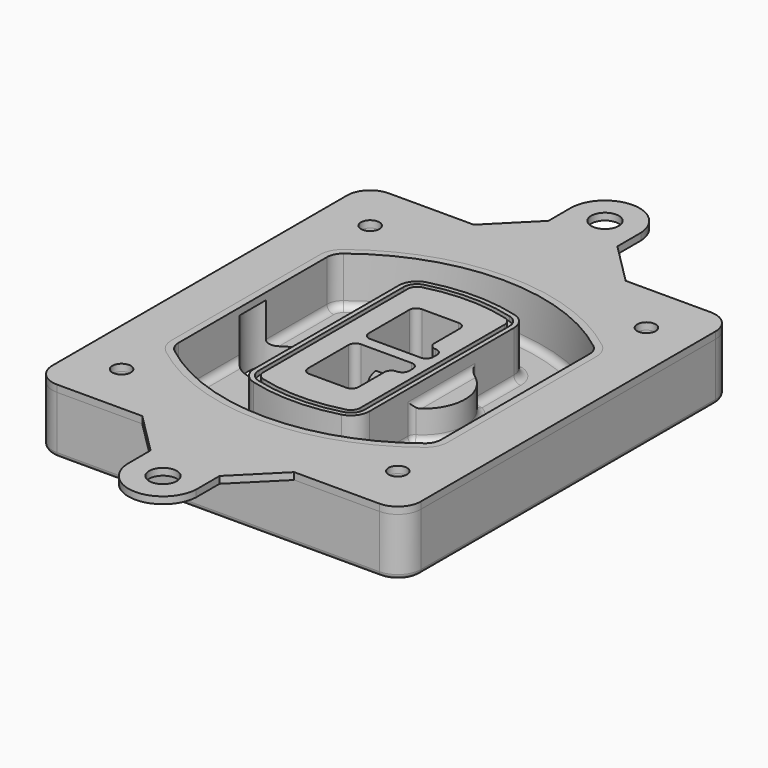
from build123d import *

# Parameters (mm, degrees)
F0_R      = 4
F1_DEPTH  = 25
F2_DEPTH  = 3
F3_DEPTH  = 18
F5_DEPTH  = 21
F6_DEPTH  = 2
F8_DEPTH  = 20
F9_DEPTH  = 16
F10_DEPTH = 25
F7_R      = 6
F7_R_2    = 4
F11_DEPTH = 6
F13_DEPTH = 9
F14_R     = 3
F15_R     = 2
F16_R     = 6
F16_R_2   = 4
F17_DEPTH = 3


with BuildPart() as f1:
    # F0 (on Top) → F1 (new body)
    with BuildSketch(Plane.XY):
        with BuildLine():
            ThreePointArc((-80, -80), (-77.0710678119, -87.0710678119), (-70, -90))
            Line((-70, -90), (70, -90))
            ThreePointArc((70, -90), (77.0710678119, -87.0710678119), (80, -80))
            Line((80, -80), (80, 80))
            ThreePointArc((80, 80), (77.0710678119, 87.0710678119), (70, 90))
            Line((70, 90), (-70, 90))
            ThreePointArc((-70, 90), (-77.0710678119, 87.0710678119), (-80, 80))
            Line((-80, 80), (-80, -80))
        make_face()
        with Locations((-60, -67.5)):
            Circle(F0_R, mode=Mode.SUBTRACT)
        with Locations((60, -67.5)):
            Circle(F0_R, mode=Mode.SUBTRACT)
        with Locations((-60, 67.5)):
            Circle(F0_R, mode=Mode.SUBTRACT)
        with BuildLine():
            ThreePointArc((-64, 40.2934422872), (-62.5820384798, 46.4328484224), (-58.6153846154, 51.3286200352))
            ThreePointArc((-58.6153846154, 51.3286200352), (0, 71.5), (58.6153846154, 51.3286200352))
            ThreePointArc((58.6153846154, 51.3286200352), (62.5820384798, 46.4328484224), (64, 40.2934422872))
            Line((64, 40.2934422872), (64, -40.2934422872))
            ThreePointArc((64, -40.2934422872), (62.5820384798, -46.4328484224), (58.6153846154, -51.3286200352))
            ThreePointArc((58.6153846154, -51.3286200352), (0, -71.5), (-58.6153846154, -51.3286200352))
            ThreePointArc((-58.6153846154, -51.3286200352), (-62.5820384798, -46.4328484224), (-64, -40.2934422872))
            Line((-64, -40.2934422872), (-64, 40.2934422872))
        make_face(mode=Mode.SUBTRACT)
        with Locations((60, 67.5)):
            Circle(F0_R, mode=Mode.SUBTRACT)
        with BuildLine():
            ThreePointArc((58.6153846154, 51.3286200352), (0, 71.5), (-58.6153846154, 51.3286200352))
            ThreePointArc((-58.6153846154, 51.3286200352), (-62.5820384798, 46.4328484224), (-64, 40.2934422872))
            Line((-64, 40.2934422872), (-64, -40.2934422872))
            ThreePointArc((-64, -40.2934422872), (-62.5820384798, -46.4328484224), (-58.6153846154, -51.3286200352))
            ThreePointArc((-58.6153846154, -51.3286200352), (0, -71.5), (58.6153846154, -51.3286200352))
            ThreePointArc((58.6153846154, -51.3286200352), (62.5820384798, -46.4328484224), (64, -40.2934422872))
            Line((64, -40.2934422872), (64, 40.2934422872))
            ThreePointArc((64, 40.2934422872), (62.5820384798, 46.4328484224), (58.6153846154, 51.3286200352))
        make_face()
        with BuildLine():
            Line((-60, -40.2934422872), (-60, 40.2934422872))
            ThreePointArc((-60, 40.2934422872), (-58.9871703427, 44.6787323838), (-56.1538461538, 48.1757121072))
            ThreePointArc((-56.1538461538, 48.1757121072), (0, 67.5), (56.1538461538, 48.1757121072))
            ThreePointArc((56.1538461538, 48.1757121072), (58.9871703427, 44.6787323838), (60, 40.2934422872))
            Line((60, 40.2934422872), (60, -40.2934422872))
            ThreePointArc((60, -40.2934422872), (58.9871703427, -44.6787323838), (56.1538461538, -48.1757121072))
            ThreePointArc((56.1538461538, -48.1757121072), (0, -67.5), (-56.1538461538, -48.1757121072))
            ThreePointArc((-56.1538461538, -48.1757121072), (-58.9871703427, -44.6787323838), (-60, -40.2934422872))
        make_face(mode=Mode.SUBTRACT)
        with BuildLine():
            ThreePointArc((-56.1538461538, 48.1757121072), (-58.9871703427, 44.6787323838), (-60, 40.2934422872))
            Line((-60, 40.2934422872), (-60, -40.2934422872))
            ThreePointArc((-60, -40.2934422872), (-58.9871703427, -44.6787323838), (-56.1538461538, -48.1757121072))
            ThreePointArc((-56.1538461538, -48.1757121072), (0, -67.5), (56.1538461538, -48.1757121072))
            ThreePointArc((56.1538461538, -48.1757121072), (58.9871703427, -44.6787323838), (60, -40.2934422872))
            Line((60, -40.2934422872), (60, 40.2934422872))
            ThreePointArc((60, 40.2934422872), (58.9871703427, 44.6787323838), (56.1538461538, 48.1757121072))
            ThreePointArc((56.1538461538, 48.1757121072), (0, 67.5), (-56.1538461538, 48.1757121072))
        make_face()
        with BuildLine():
            ThreePointArc((54.3076923077, 45.8110311612), (56.2910192399, 43.3631453548), (57, 40.2934422872))
            Line((57, 40.2934422872), (57, -40.2934422872))
            ThreePointArc((57, -40.2934422872), (56.2910192399, -43.3631453548), (54.3076923077, -45.8110311612))
            ThreePointArc((54.3076923077, -45.8110311612), (0, -64.5), (-54.3076923077, -45.8110311612))
            ThreePointArc((-54.3076923077, -45.8110311612), (-56.2910192399, -43.3631453548), (-57, -40.2934422872))
            Line((-57, -40.2934422872), (-57, 40.2934422872))
            ThreePointArc((-57, 40.2934422872), (-56.2910192399, 43.3631453548), (-54.3076923077, 45.8110311612))
            ThreePointArc((-54.3076923077, 45.8110311612), (0, 64.5), (54.3076923077, 45.8110311612))
        make_face(mode=Mode.SUBTRACT)
        with BuildLine():
            Line((57, -40.2934422872), (57, 40.2934422872))
            ThreePointArc((57, 40.2934422872), (56.2910192399, 43.3631453548), (54.3076923077, 45.8110311612))
            ThreePointArc((54.3076923077, 45.8110311612), (0, 64.5), (-54.3076923077, 45.8110311612))
            ThreePointArc((-54.3076923077, 45.8110311612), (-56.2910192399, 43.3631453548), (-57, 40.2934422872))
            Line((-57, 40.2934422872), (-57, -40.2934422872))
            ThreePointArc((-57, -40.2934422872), (-56.2910192399, -43.3631453548), (-54.3076923077, -45.8110311612))
            ThreePointArc((-54.3076923077, -45.8110311612), (0, -64.5), (54.3076923077, -45.8110311612))
            ThreePointArc((54.3076923077, -45.8110311612), (56.2910192399, -43.3631453548), (57, -40.2934422872))
        make_face()
    extrude(amount=-F1_DEPTH)

    # F0 (on Top) → F2 (join)
    with BuildSketch(Plane.XY):
        with BuildLine():
            ThreePointArc((-56.1538461538, 48.1757121072), (-58.9871703427, 44.6787323838), (-60, 40.2934422872))
            Line((-60, 40.2934422872), (-60, -40.2934422872))
            ThreePointArc((-60, -40.2934422872), (-58.9871703427, -44.6787323838), (-56.1538461538, -48.1757121072))
            ThreePointArc((-56.1538461538, -48.1757121072), (0, -67.5), (56.1538461538, -48.1757121072))
            ThreePointArc((56.1538461538, -48.1757121072), (58.9871703427, -44.6787323838), (60, -40.2934422872))
            Line((60, -40.2934422872), (60, 40.2934422872))
            ThreePointArc((60, 40.2934422872), (58.9871703427, 44.6787323838), (56.1538461538, 48.1757121072))
            ThreePointArc((56.1538461538, 48.1757121072), (0, 67.5), (-56.1538461538, 48.1757121072))
        make_face()
        with BuildLine():
            ThreePointArc((54.3076923077, 45.8110311612), (56.2910192399, 43.3631453548), (57, 40.2934422872))
            Line((57, 40.2934422872), (57, -40.2934422872))
            ThreePointArc((57, -40.2934422872), (56.2910192399, -43.3631453548), (54.3076923077, -45.8110311612))
            ThreePointArc((54.3076923077, -45.8110311612), (0, -64.5), (-54.3076923077, -45.8110311612))
            ThreePointArc((-54.3076923077, -45.8110311612), (-56.2910192399, -43.3631453548), (-57, -40.2934422872))
            Line((-57, -40.2934422872), (-57, 40.2934422872))
            ThreePointArc((-57, 40.2934422872), (-56.2910192399, 43.3631453548), (-54.3076923077, 45.8110311612))
            ThreePointArc((-54.3076923077, 45.8110311612), (0, 64.5), (54.3076923077, 45.8110311612))
        make_face(mode=Mode.SUBTRACT)
    extrude(amount=F2_DEPTH)

    # F0 (on Top) → F3 (cut)
    with BuildSketch(Plane.XY):
        with BuildLine():
            Line((57, -40.2934422872), (57, 40.2934422872))
            ThreePointArc((57, 40.2934422872), (56.2910192399, 43.3631453548), (54.3076923077, 45.8110311612))
            ThreePointArc((54.3076923077, 45.8110311612), (0, 64.5), (-54.3076923077, 45.8110311612))
            ThreePointArc((-54.3076923077, 45.8110311612), (-56.2910192399, 43.3631453548), (-57, 40.2934422872))
            Line((-57, 40.2934422872), (-57, -40.2934422872))
            ThreePointArc((-57, -40.2934422872), (-56.2910192399, -43.3631453548), (-54.3076923077, -45.8110311612))
            ThreePointArc((-54.3076923077, -45.8110311612), (0, -64.5), (54.3076923077, -45.8110311612))
            ThreePointArc((54.3076923077, -45.8110311612), (56.2910192399, -43.3631453548), (57, -40.2934422872))
        make_face()
    extrude(amount=-F3_DEPTH, mode=Mode.SUBTRACT)

    # F4 (on face) → F5 (join, through all)
    with BuildSketch(Plane.XY.offset(3)):
        with BuildLine():
            ThreePointArc((-25, -39.2465276821), (-23.3511545998, -44.1109737193), (-19.0842911877, -46.9702398883))
            ThreePointArc((-19.0842911877, -46.9702398883), (0, -49.5), (19.0842911877, -46.9702398883))
            ThreePointArc((19.0842911877, -46.9702398883), (23.3511545998, -44.1109737193), (25, -39.2465276821))
            Line((25, -39.2465276821), (25, 39.2465276821))
            ThreePointArc((25, 39.2465276821), (23.3511545998, 44.1109737193), (19.0842911877, 46.9702398883))
            ThreePointArc((19.0842911877, 46.9702398883), (0, 49.5), (-19.0842911877, 46.9702398883))
            ThreePointArc((-19.0842911877, 46.9702398883), (-23.3511545998, 44.1109737193), (-25, 39.2465276821))
            Line((-25, 39.2465276821), (-25, -39.2465276821))
        make_face()
        with BuildLine():
            ThreePointArc((18.5632183908, 45.0393118368), (21.7633659499, 42.89486221), (23, 39.2465276821))
            Line((23, 39.2465276821), (23, -39.2465276821))
            ThreePointArc((23, -39.2465276821), (21.7633659499, -42.89486221), (18.5632183908, -45.0393118368))
            ThreePointArc((18.5632183908, -45.0393118368), (0, -47.5), (-18.5632183908, -45.0393118368))
            ThreePointArc((-18.5632183908, -45.0393118368), (-21.7633659499, -42.89486221), (-23, -39.2465276821))
            Line((-23, -39.2465276821), (-23, 39.2465276821))
            ThreePointArc((-23, 39.2465276821), (-21.7633659499, 42.89486221), (-18.5632183908, 45.0393118368))
            ThreePointArc((-18.5632183908, 45.0393118368), (0, 47.5), (18.5632183908, 45.0393118368))
        make_face(mode=Mode.SUBTRACT)
        with BuildLine():
            Line((23, -39.2465276821), (23, 39.2465276821))
            ThreePointArc((23, 39.2465276821), (21.7633659499, 42.89486221), (18.5632183908, 45.0393118368))
            ThreePointArc((18.5632183908, 45.0393118368), (0, 47.5), (-18.5632183908, 45.0393118368))
            ThreePointArc((-18.5632183908, 45.0393118368), (-21.7633659499, 42.89486221), (-23, 39.2465276821))
            Line((-23, 39.2465276821), (-23, -39.2465276821))
            ThreePointArc((-23, -39.2465276821), (-21.7633659499, -42.89486221), (-18.5632183908, -45.0393118368))
            ThreePointArc((-18.5632183908, -45.0393118368), (0, -47.5), (18.5632183908, -45.0393118368))
            ThreePointArc((18.5632183908, -45.0393118368), (21.7633659499, -42.89486221), (23, -39.2465276821))
        make_face()
        with BuildLine():
            ThreePointArc((18.0421455939, 43.1083837852), (20.1755772999, 41.6787507007), (21, 39.2465276821))
            Line((21, 39.2465276821), (21, -39.2465276821))
            ThreePointArc((21, -39.2465276821), (20.1755772999, -41.6787507007), (18.0421455939, -43.1083837852))
            ThreePointArc((18.0421455939, -43.1083837852), (0, -45.5), (-18.0421455939, -43.1083837852))
            ThreePointArc((-18.0421455939, -43.1083837852), (-20.1755772999, -41.6787507007), (-21, -39.2465276821))
            Line((-21, -39.2465276821), (-21, 39.2465276821))
            ThreePointArc((-21, 39.2465276821), (-20.1755772999, 41.6787507007), (-18.0421455939, 43.1083837852))
            ThreePointArc((-18.0421455939, 43.1083837852), (0, 45.5), (18.0421455939, 43.1083837852))
        make_face(mode=Mode.SUBTRACT)
        with BuildLine():
            Line((21, -39.2465276821), (21, 39.2465276821))
            ThreePointArc((21, 39.2465276821), (20.1755772999, 41.6787507007), (18.0421455939, 43.1083837852))
            ThreePointArc((18.0421455939, 43.1083837852), (0, 45.5), (-18.0421455939, 43.1083837852))
            ThreePointArc((-18.0421455939, 43.1083837852), (-20.1755772999, 41.6787507007), (-21, 39.2465276821))
            Line((-21, 39.2465276821), (-21, -39.2465276821))
            ThreePointArc((-21, -39.2465276821), (-20.1755772999, -41.6787507007), (-18.0421455939, -43.1083837852))
            ThreePointArc((-18.0421455939, -43.1083837852), (0, -45.5), (18.0421455939, -43.1083837852))
            ThreePointArc((18.0421455939, -43.1083837852), (20.1755772999, -41.6787507007), (21, -39.2465276821))
        make_face()
        with BuildLine():
            Line((-8, -2.5), (14, -2.5))
            ThreePointArc((14, -2.5), (16.1213203436, -3.3786796564), (17, -5.5))
            Line((17, -5.5), (17, -7.5))
            ThreePointArc((17, -7.5), (16.1213203436, -9.6213203436), (14, -10.5))
            ThreePointArc((14, -10.5), (11.8786796564, -11.3786796564), (11, -13.5))
            Line((11, -13.5), (11, -27.5))
            ThreePointArc((11, -27.5), (10.1213203436, -29.6213203436), (8, -30.5))
            Line((8, -30.5), (-8, -30.5))
            ThreePointArc((-8, -30.5), (-10.1213203436, -29.6213203436), (-11, -27.5))
            Line((-11, -27.5), (-11, -5.5))
            ThreePointArc((-11, -5.5), (-10.1213203436, -3.3786796564), (-8, -2.5))
        make_face(mode=Mode.SUBTRACT)
        with BuildLine():
            ThreePointArc((-8, 2.5), (-10.1213203436, 3.3786796564), (-11, 5.5))
            Line((-11, 5.5), (-11, 27.5))
            ThreePointArc((-11, 27.5), (-10.1213203436, 29.6213203436), (-8, 30.5))
            Line((-8, 30.5), (8, 30.5))
            ThreePointArc((8, 30.5), (10.1213203436, 29.6213203436), (11, 27.5))
            Line((11, 27.5), (11, 13.5))
            ThreePointArc((11, 13.5), (11.8786796564, 11.3786796564), (14, 10.5))
            ThreePointArc((14, 10.5), (16.1213203436, 9.6213203436), (17, 7.5))
            Line((17, 7.5), (17, 5.5))
            ThreePointArc((17, 5.5), (16.1213203436, 3.3786796564), (14, 2.5))
            Line((14, 2.5), (-8, 2.5))
        make_face(mode=Mode.SUBTRACT)
    extrude(amount=-F5_DEPTH)

    # F4 (on face) → F6 (cut)
    with BuildSketch(Plane.XY.offset(3)):
        with BuildLine():
            Line((23, -39.2465276821), (23, 39.2465276821))
            ThreePointArc((23, 39.2465276821), (21.7633659499, 42.89486221), (18.5632183908, 45.0393118368))
            ThreePointArc((18.5632183908, 45.0393118368), (0, 47.5), (-18.5632183908, 45.0393118368))
            ThreePointArc((-18.5632183908, 45.0393118368), (-21.7633659499, 42.89486221), (-23, 39.2465276821))
            Line((-23, 39.2465276821), (-23, -39.2465276821))
            ThreePointArc((-23, -39.2465276821), (-21.7633659499, -42.89486221), (-18.5632183908, -45.0393118368))
            ThreePointArc((-18.5632183908, -45.0393118368), (0, -47.5), (18.5632183908, -45.0393118368))
            ThreePointArc((18.5632183908, -45.0393118368), (21.7633659499, -42.89486221), (23, -39.2465276821))
        make_face()
        with BuildLine():
            ThreePointArc((18.0421455939, 43.1083837852), (20.1755772999, 41.6787507007), (21, 39.2465276821))
            Line((21, 39.2465276821), (21, -39.2465276821))
            ThreePointArc((21, -39.2465276821), (20.1755772999, -41.6787507007), (18.0421455939, -43.1083837852))
            ThreePointArc((18.0421455939, -43.1083837852), (0, -45.5), (-18.0421455939, -43.1083837852))
            ThreePointArc((-18.0421455939, -43.1083837852), (-20.1755772999, -41.6787507007), (-21, -39.2465276821))
            Line((-21, -39.2465276821), (-21, 39.2465276821))
            ThreePointArc((-21, 39.2465276821), (-20.1755772999, 41.6787507007), (-18.0421455939, 43.1083837852))
            ThreePointArc((-18.0421455939, 43.1083837852), (0, 45.5), (18.0421455939, 43.1083837852))
        make_face(mode=Mode.SUBTRACT)
    extrude(amount=-F6_DEPTH, mode=Mode.SUBTRACT)

    # F7 (on face) → F8 (join)
    with BuildSketch(Plane(origin=(0, 0, -25), x_dir=(1, 0, 0), z_dir=(0, 0, -1))):
        with BuildLine():
            ThreePointArc((3.28842436, 0), (16.7567035675, 13.4682792075), (30.224982775, 0))
            Line((30.224982775, 0), (35.224982775, 0))
            ThreePointArc((35.224982775, 0), (16.7567035675, 18.4682792075), (-1.71157564, 0))
            Line((-1.71157564, 0), (3.28842436, 0))
        make_face()
        with BuildLine():
            Line((3.28842436, 0), (30.224982775, 0))
            ThreePointArc((30.224982775, 0), (16.7567035675, 13.4682792075), (3.28842436, 0))
        make_face()
        with BuildLine():
            ThreePointArc((3.28842436, 0), (16.7567035675, -13.4682792075), (30.224982775, 0))
            Line((30.224982775, 0), (3.28842436, 0))
        make_face()
        with BuildLine():
            Line((35.224982775, 0), (30.224982775, 0))
            ThreePointArc((30.224982775, 0), (16.7567035675, -13.4682792075), (3.28842436, 0))
            Line((3.28842436, 0), (-1.71157564, 0))
            ThreePointArc((-1.71157564, 0), (16.7567035675, -18.4682792075), (35.224982775, 0))
        make_face()
    extrude(amount=-F8_DEPTH)

    # F7 (on face) → F9 (cut)
    with BuildSketch(Plane(origin=(0, 0, -25), x_dir=(1, 0, 0), z_dir=(0, 0, -1))):
        with BuildLine():
            Line((3.28842436, 0), (30.224982775, 0))
            ThreePointArc((30.224982775, 0), (16.7567035675, 13.4682792075), (3.28842436, 0))
        make_face()
        with BuildLine():
            ThreePointArc((3.28842436, 0), (16.7567035675, -13.4682792075), (30.224982775, 0))
            Line((30.224982775, 0), (3.28842436, 0))
        make_face()
    extrude(amount=-F9_DEPTH, mode=Mode.SUBTRACT)

    # F7 (on face) → F10 (cut)
    with BuildSketch(Plane(origin=(0, 0, -25), x_dir=(1, 0, 0), z_dir=(0, 0, -1))):
        with BuildLine():
            Line((-59.0318229325, 0), (-32.0952645175, 0))
            ThreePointArc((-32.0952645175, 0), (-45.563543725, 13.4682792075), (-59.0318229325, 0))
        make_face()
        with BuildLine():
            ThreePointArc((-59.0318229325, 0), (-45.563543725, -13.4682792075), (-32.0952645175, 0))
            Line((-32.0952645175, 0), (-59.0318229325, 0))
        make_face()
    extrude(amount=-F10_DEPTH, mode=Mode.SUBTRACT)

    # F7 (on face) → F11 (cut)
    with BuildSketch(Plane(origin=(0, 0, -25), x_dir=(1, 0, 0), z_dir=(0, 0, -1))):
        with Locations((60, -67.5)):
            Circle(F7_R)
        with Locations((60, -67.5)):
            Circle(F7_R_2, mode=Mode.SUBTRACT)
        with Locations((-60, -67.5)):
            Circle(F7_R)
        with Locations((-60, -67.5)):
            Circle(F7_R_2, mode=Mode.SUBTRACT)
        with Locations((-60, 67.5)):
            Circle(F7_R)
        with Locations((-60, 67.5)):
            Circle(F7_R_2, mode=Mode.SUBTRACT)
        with Locations((60, 67.5)):
            Circle(F7_R)
        with Locations((60, 67.5)):
            Circle(F7_R_2, mode=Mode.SUBTRACT)
    extrude(amount=-F11_DEPTH, mode=Mode.SUBTRACT)

    # F12 (on face) → F13 (cut, through all)
    with BuildSketch(Plane(origin=(0, 0, -9), x_dir=(1, 0, 0), z_dir=(0, 0, -1))):
        with BuildLine():
            Line((11, 13.5), (11, 17.5481537753))
            ThreePointArc((11, 17.5481537753), (2.5696536419, 11.8239143813), (-1.5415842455, 2.5))
            Line((-1.5415842455, 2.5), (3.5224848595, 2.5))
            ThreePointArc((3.5224848595, 2.5), (6.1857188154, 8.3455872281), (11.2536447004, 12.2927168648))
            ThreePointArc((11.2536447004, 12.2927168648), (11.0640958889, 12.8831798879), (11, 13.5))
        make_face()
        with BuildLine():
            ThreePointArc((11.2536447004, -12.2927168648), (6.1857188154, -8.3455872281), (3.5224848595, -2.5))
            Line((3.5224848595, -2.5), (-1.5415842455, -2.5))
            ThreePointArc((-1.5415842455, -2.5), (2.5696536419, -11.8239143813), (11, -17.5481537753))
            Line((11, -17.5481537753), (11, -13.5))
            ThreePointArc((11, -13.5), (11.0640958889, -12.8831798879), (11.2536447004, -12.2927168648))
        make_face()
        with BuildLine():
            ThreePointArc((11.2536447004, 12.2927168648), (6.1857188154, 8.3455872281), (3.5224848595, 2.5))
            Line((3.5224848595, 2.5), (14, 2.5))
            ThreePointArc((14, 2.5), (16.1213203436, 3.3786796564), (17, 5.5))
            Line((17, 5.5), (17, 7.5))
            ThreePointArc((17, 7.5), (16.1213203436, 9.6213203436), (14, 10.5))
            ThreePointArc((14, 10.5), (12.3601599782, 10.9878446101), (11.2536447004, 12.2927168648))
        make_face()
        with BuildLine():
            Line((14, -2.5), (3.5224848595, -2.5))
            ThreePointArc((3.5224848595, -2.5), (6.1857188154, -8.3455872281), (11.2536447004, -12.2927168648))
            ThreePointArc((11.2536447004, -12.2927168648), (12.3601599782, -10.9878446101), (14, -10.5))
            ThreePointArc((14, -10.5), (16.1213203436, -9.6213203436), (17, -7.5))
            Line((17, -7.5), (17, -5.5))
            ThreePointArc((17, -5.5), (16.1213203436, -3.3786796564), (14, -2.5))
        make_face()
    extrude(amount=F13_DEPTH, mode=Mode.SUBTRACT)

    # F14
    f14_edges = [f1.edges().sort_by_distance(p)[0] for p in [
        (-57, -23.703476, -18),
        (-57, 23.703476, -18),
        (25, 0, -5),
        (25, 16.526506, -11.5),
        (25, -16.526506, -11.5),
        (25, -27.886517, -18),
        (35.224983, 0, -18),
    ]]
    fillet(f14_edges, radius=F14_R)

    # F15
    f15_edges = [f1.edges().sort_by_distance(p)[0] for p in [
        (0, -90, -25),
    ]]
    fillet(f15_edges, radius=F15_R)


with BuildPart() as f17:
    # F16 (on face) → F17 (new body, through all)
    with BuildSketch(Plane.XY):
        with BuildLine():
            Line((32.9778034812, -90), (-33, -90))
            Line((-33, -90), (-15, -108))
            Line((-15, -108), (-15, -120))
            ThreePointArc((-15, -120), (-0.4080121214, -134.9944498435), (14.9778034812, -120.8157223053))
            Line((14.9778034812, -120.8157223053), (14.9778034812, -108))
            Line((14.9778034812, -108), (32.9778034812, -90))
        make_face()
        with Locations((0, -120)):
            Circle(F16_R, mode=Mode.SUBTRACT)
        with BuildLine():
            Line((32.9778034812, 90), (-33, 90))
            Line((-33, 90), (-70, 90))
            ThreePointArc((-70, 90), (-77.0710678119, 87.0710678119), (-80, 80))
            Line((-80, 80), (-80, -80))
            ThreePointArc((-80, -80), (-77.0710678119, -87.0710678119), (-70, -90))
            Line((-70, -90), (-33, -90))
            Line((-33, -90), (32.9778034812, -90))
            Line((32.9778034812, -90), (70, -90))
            ThreePointArc((70, -90), (77.0710678119, -87.0710678119), (80, -80))
            Line((80, -80), (80, 80))
            ThreePointArc((80, 80), (77.0710678119, 87.0710678119), (70, 90))
            Line((70, 90), (32.9778034812, 90))
        make_face()
        with Locations((-60, -67.5)):
            Circle(F16_R_2, mode=Mode.SUBTRACT)
        with Locations((60, -67.5)):
            Circle(F16_R_2, mode=Mode.SUBTRACT)
        with BuildLine():
            ThreePointArc((-60, 40.2934422872), (-58.9871703427, 44.6787323838), (-56.1538461538, 48.1757121072))
            ThreePointArc((-56.1538461538, 48.1757121072), (0, 67.5), (56.1538461538, 48.1757121072))
            ThreePointArc((56.1538461538, 48.1757121072), (58.9871703427, 44.6787323838), (60, 40.2934422872))
            Line((60, 40.2934422872), (60, -40.2934422872))
            ThreePointArc((60, -40.2934422872), (58.9871703427, -44.6787323838), (56.1538461538, -48.1757121072))
            ThreePointArc((56.1538461538, -48.1757121072), (0, -67.5), (-56.1538461538, -48.1757121072))
            ThreePointArc((-56.1538461538, -48.1757121072), (-58.9871703427, -44.6787323838), (-60, -40.2934422872))
            Line((-60, -40.2934422872), (-60, 40.2934422872))
        make_face(mode=Mode.SUBTRACT)
        with Locations((-60, 67.5)):
            Circle(F16_R_2, mode=Mode.SUBTRACT)
        with Locations((60, 67.5)):
            Circle(F16_R_2, mode=Mode.SUBTRACT)
        with BuildLine():
            Line((-15, 108), (-33, 90))
            Line((-33, 90), (32.9778034812, 90))
            Line((32.9778034812, 90), (14.9778034812, 108))
            Line((14.9778034812, 108), (14.9778034812, 120.8157223053))
            ThreePointArc((14.9778034812, 120.8157223053), (-0.4080121214, 134.9944498435), (-15, 120))
            Line((-15, 120), (-15, 108))
        make_face()
        with Locations((0, 120)):
            Circle(F16_R, mode=Mode.SUBTRACT)
    extrude(amount=F17_DEPTH)


solid = Compound([f1.part, f17.part])
